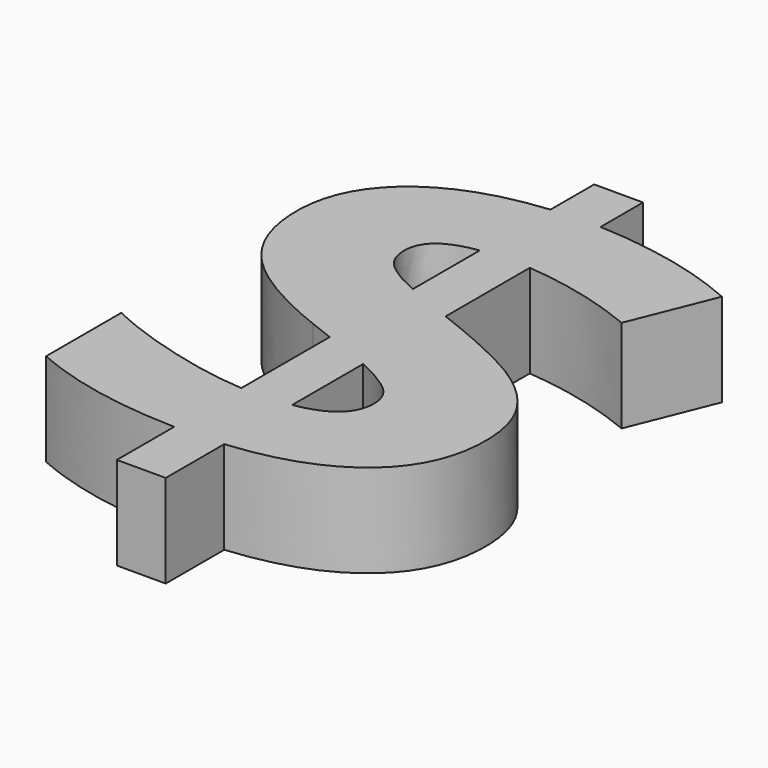
from build123d import *

# Parameters (mm, degrees)
F0_TEXT_SIZE = 78.5135711771
F1_DEPTH     = 10


# Not quite as in the source:
# - Text() gives the source's letters only with a copy of the font that has no kerning and outlines rounded to 1/6400 em; it was checked with that copy


with BuildPart() as f1:
    # F0 (on Top) → F1 (new body)
    with BuildSketch(Plane.XY):
        with Locations((0, 0)):
            Text('$', F0_TEXT_SIZE, font='Open Sans', font_style=FontStyle.BOLD, text_align=(TextAlign.LEFT, TextAlign.BOTTOM))
    extrude(amount=F1_DEPTH)


solid = f1.part
